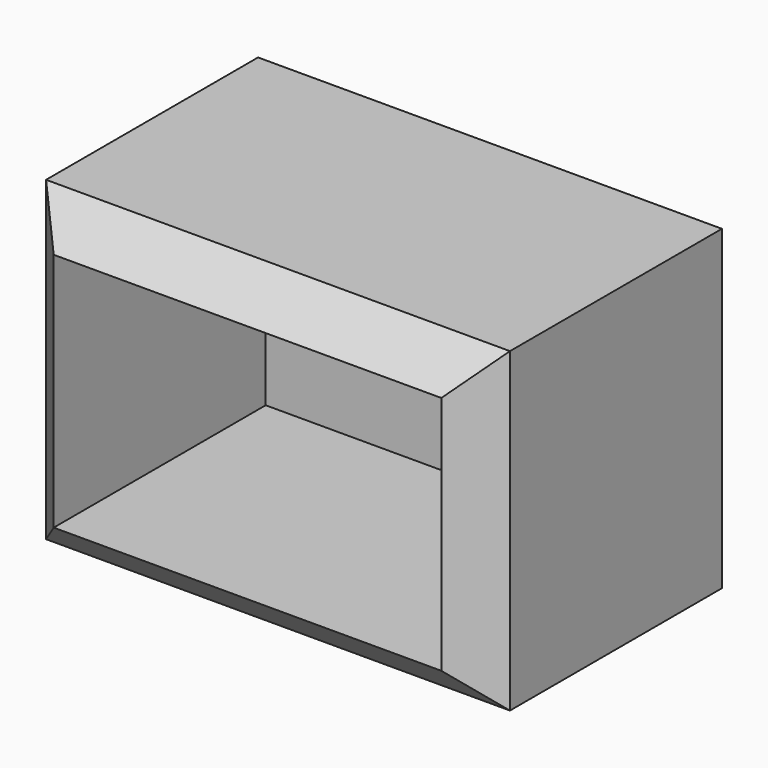
from build123d import *

# Parameters (mm, degrees)
F0_W     = 61.8086736649
F0_H     = 40.3841938823
F1_DEPTH = 42.164
F2_T     = -5.08
F3_SIZE  = 5.07999
F4_SIZE  = 5.07999
F5_SIZE  = 5.07999


# Not quite as in the source:
# - a fillet or chamfer is up to 0.001 mm smaller than in the source, because OpenCascade refuses the exact size


with BuildPart() as f1:
    # F0 (on Top) → F1 (new body)
    with BuildSketch(Plane.XY):
        with Locations((-2.8439583257, 1.9907699898)):
            Rectangle(F0_W, F0_H)
    extrude(amount=F1_DEPTH)

    # F2
    f2_openings = [f1.faces().sort_by_distance(p)[0] for p in [
        (-2.843958, -18.201327, 21.082),
    ]]
    offset(amount=F2_T, openings=f2_openings)

    # F3 (size 5.08 in the source; OpenCascade refuses exactly that, so slightly less here)
    f3_edges = [f1.edges().sort_by_distance(p)[0] for p in [
        (-2.843958, -18.201327, 42.164),
    ]]
    chamfer(f3_edges, length=F3_SIZE)

    # F4 (size 5.08 in the source; OpenCascade refuses exactly that, so slightly less here)
    f4_edges = [f1.edges().sort_by_distance(p)[0] for p in [
        (-33.748295, -18.201327, 18.542005),
        (28.060379, -18.201327, 18.542005),
    ]]
    chamfer(f4_edges, length=F4_SIZE)

    # F5 (size 5.08 in the source; OpenCascade refuses exactly that, so slightly less here)
    f5_edges = [f1.edges().sort_by_distance(p)[0] for p in [
        (-2.843958, -18.201327, 0),
    ]]
    chamfer(f5_edges, length=F5_SIZE)


solid = f1.part
